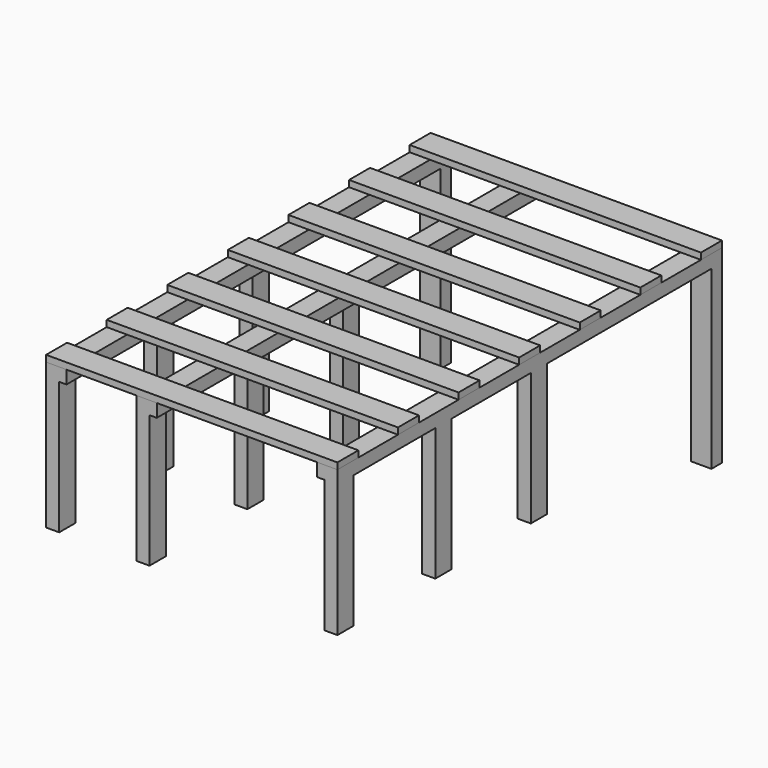
from build123d import *

# Parameters (mm, degrees)
F0_W     = 70
F0_H     = 1650
F1_DEPTH = 45
F2_W     = 45
F2_H     = 70
F3_DEPTH = 455
F2_W_2   = 70
F2_H_2   = 45
F4_DEPTH = 605
F5_W     = 70
F5_H     = 90
F5_W_2   = 930
F6_DEPTH = 22


# Not quite as in the source:
# - a feature names something its author has since deleted; it is built from what else it names


with BuildPart() as f1:
    # F0 (on Top) → F1 (new body)
    with BuildSketch(Plane.XY):
        with Locations((0, -825)):
            Rectangle(F0_W, F0_H)
    extrude(amount=F1_DEPTH)

    # F2 (on face) → F3, piece 2 (join)
    with BuildSketch(Plane(origin=(0, 0, 0), x_dir=(1, 0, 0), z_dir=(0, 0, -1))):
        with Locations((-12.5, 785)):
            Rectangle(F2_W, F2_H)
        with Locations((-12.5, 1615)):
            Rectangle(F2_W, F2_H)
        with Locations((-12.5, 1195)):
            Rectangle(F2_W, F2_H)
    extrude(amount=F3_DEPTH)


with BuildPart() as f1b:
    # F0 (on Top) → F1, piece 2 (new body)
    with BuildSketch(Plane.XY):
        with Locations((620, -825)):
            Rectangle(F0_W, F0_H)
    extrude(amount=F1_DEPTH)

    # F2 (on face) → F3, piece 3 (join)
    with BuildSketch(Plane(origin=(0, 0, 0), x_dir=(1, 0, 0), z_dir=(0, 0, -1))):
        with Locations((632.5, 1615)):
            Rectangle(F2_W, F2_H)
        with Locations((632.5, 785)):
            Rectangle(F2_W, F2_H)
        with Locations((632.5, 1195)):
            Rectangle(F2_W, F2_H)
    extrude(amount=F3_DEPTH)

    # F2 (on face) → F4 (join)
    with BuildSketch(Plane(origin=(0, 0, 0), x_dir=(1, 0, 0), z_dir=(0, 0, -1))):
        with Locations((620, 22.5)):
            Rectangle(F2_W_2, F2_H_2)
    extrude(amount=F4_DEPTH)


with BuildPart() as f1c:
    # F0 (on Top) → F1, piece 3 (new body)
    with BuildSketch(Plane.XY):
        with Locations((-310, -825)):
            Rectangle(F0_W, F0_H)
    extrude(amount=F1_DEPTH)

    # F2 (on face) → F3 (join)
    with BuildSketch(Plane(origin=(0, 0, 0), x_dir=(1, 0, 0), z_dir=(0, 0, -1))):
        with Locations((-322.5, 785)):
            Rectangle(F2_W, F2_H)
        with Locations((-322.5, 1615)):
            Rectangle(F2_W, F2_H)
        with Locations((-322.5, 1195)):
            Rectangle(F2_W, F2_H)
    extrude(amount=F3_DEPTH)

    # F2 (on face) → F4, piece 2 (join)
    with BuildSketch(Plane(origin=(0, 0, 0), x_dir=(1, 0, 0), z_dir=(0, 0, -1))):
        with Locations((-310, 22.5)):
            Rectangle(F2_W_2, F2_H_2)
    extrude(amount=F4_DEPTH)


with BuildPart() as f6:
    # F5 (on face) → F6 (new body)
    with BuildSketch(Plane.XY.offset(45)):
        with Locations((-310, -1605)):
            Rectangle(F5_W, F5_H)
        with Locations((190, -1605)):
            Rectangle(F5_W_2, F5_H)
    extrude(amount=F6_DEPTH)


with BuildPart() as f6b:
    # F5 (on face) → F6, piece 2 (new body)
    with BuildSketch(Plane.XY.offset(45)):
        with Locations((-310, -1345)):
            Rectangle(F5_W, F5_H)
        with Locations((190, -1345)):
            Rectangle(F5_W_2, F5_H)
    extrude(amount=F6_DEPTH)


with BuildPart() as f6c:
    # F5 (on face) → F6, piece 3 (new body)
    with BuildSketch(Plane.XY.offset(45)):
        with Locations((-310, -1085)):
            Rectangle(F5_W, F5_H)
        with Locations((190, -1085)):
            Rectangle(F5_W_2, F5_H)
    extrude(amount=F6_DEPTH)


with BuildPart() as f6d:
    # F5 (on face) → F6, piece 4 (new body)
    with BuildSketch(Plane.XY.offset(45)):
        with Locations((-310, -825)):
            Rectangle(F5_W, F5_H)
        with Locations((190, -825)):
            Rectangle(F5_W_2, F5_H)
    extrude(amount=F6_DEPTH)


with BuildPart() as f6e:
    # F5 (on face) → F6, piece 5 (new body)
    with BuildSketch(Plane.XY.offset(45)):
        with Locations((-310, -565)):
            Rectangle(F5_W, F5_H)
        with Locations((190, -565)):
            Rectangle(F5_W_2, F5_H)
    extrude(amount=F6_DEPTH)


with BuildPart() as f6f:
    # F5 (on face) → F6, piece 6 (new body)
    with BuildSketch(Plane.XY.offset(45)):
        with Locations((-310, -305)):
            Rectangle(F5_W, F5_H)
        with Locations((190, -305)):
            Rectangle(F5_W_2, F5_H)
    extrude(amount=F6_DEPTH)


with BuildPart() as f6g:
    # F5 (on face) → F6, piece 7 (new body)
    with BuildSketch(Plane.XY.offset(45)):
        with Locations((-310, -45)):
            Rectangle(F5_W, F5_H)
        with Locations((190, -45)):
            Rectangle(F5_W_2, F5_H)
    extrude(amount=F6_DEPTH)


solid = Compound([f1.part, f1b.part, f1c.part, f6.part, f6b.part, f6c.part, f6d.part, f6e.part, f6f.part, f6g.part])
